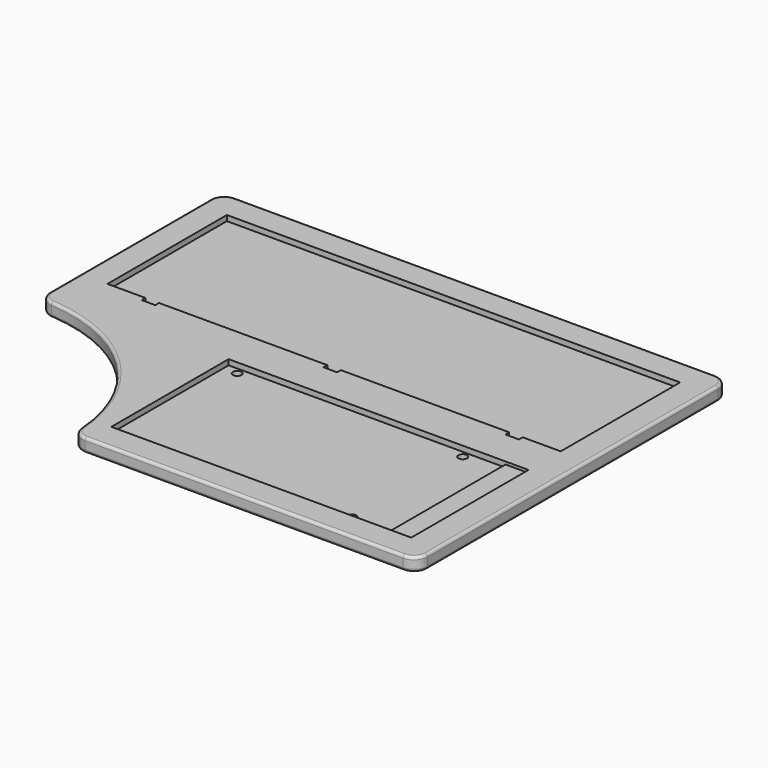
from build123d import *

# Parameters (mm, degrees)
F1_DEPTH = 5
F0_W     = 102
F0_H     = 54
F0_R     = 1.6
F2_DEPTH = 3
F0_W_2   = 8.5
F3_DEPTH = 4
F4_R     = 5
F5_R     = 1


with BuildPart() as f1:
    # F0 (on Top) → F1 (new body)
    with BuildSketch(Plane.XY):
        with BuildLine():
            Line((93.8627476096, 86.3866787127), (-93.1372523904, 86.3866787127))
            Line((-93.1372523904, 86.3866787127), (-93.1372523904, 2.5552856157))
            ThreePointArc((-93.1372523904, 2.5552856157), (-50.7122317842, -15.0177333034), (-33.1392128652, -57.4427539095))
            Line((-33.1392128652, -57.4427539095), (93.8627476096, -57.4427539095))
            Line((93.8627476096, -57.4427539095), (93.8627476096, 86.3866787127))
        make_face()
        Polygon((-26.6372523904, -47.4427539095), (-26.6372523904, 6.5572460905), (75.3627476096, 6.5572460905), (83.8627476096, 6.5572460905), (83.8627476096, -47.4427539095), (75.3627476096, -47.4427539095), align=None, mode=Mode.SUBTRACT)
        Polygon((-83.1372523904, 21.3866787127), (-83.1372523904, 76.3866787127), (83.8627476096, 76.3866787127), (83.8627476096, 21.3866787127), (69.8627476096, 21.3866787127), (69.8627476096, 19.6525212377), (64.8627476096, 19.6525212377), (64.8627476096, 21.3866787127), (2.8627476096, 21.3866787127), (2.8627476096, 19.6525212377), (-2.1372523904, 19.6525212377), (-2.1372523904, 21.3866787127), (-64.1372523904, 21.3866787127), (-64.1372523904, 19.6525212377), (-69.1372523904, 19.6525212377), (-69.1372523904, 21.3866787127), align=None, mode=Mode.SUBTRACT)
    extrude(amount=F1_DEPTH)

    # F0 (on Top) → F2 (join)
    with BuildSketch(Plane.XY):
        Polygon((83.8627476096, 76.3866787127), (-83.1372523904, 76.3866787127), (-83.1372523904, 21.3866787127), (-69.1372523904, 21.3866787127), (-69.1372523904, 19.6525212377), (-64.1372523904, 19.6525212377), (-64.1372523904, 21.3866787127), (-2.1372523904, 21.3866787127), (-2.1372523904, 19.6525212377), (2.8627476096, 19.6525212377), (2.8627476096, 21.3866787127), (64.8627476096, 21.3866787127), (64.8627476096, 19.6525212377), (69.8627476096, 19.6525212377), (69.8627476096, 21.3866787127), (83.8627476096, 21.3866787127), align=None)
        with Locations((24.3627476096, -20.4427539095)):
            Rectangle(F0_W, F0_H)
        with Locations((-21.5372523904, 4.1572460905)):
            Circle(F0_R, mode=Mode.SUBTRACT)
        with Locations((60.0627476096, -45.0427539095)):
            Circle(F0_R, mode=Mode.SUBTRACT)
        with Locations((61.5627476096, 4.1572460905)):
            Circle(F0_R, mode=Mode.SUBTRACT)
    extrude(amount=F2_DEPTH)

    # F0 (on Top) → F3 (join)
    with BuildSketch(Plane.XY):
        with Locations((79.6127476096, -20.4427539095)):
            Rectangle(F0_W_2, F0_H)
    extrude(amount=F3_DEPTH)

    # F4
    f4_edges = [f1.edges().sort_by_distance(p)[0] for p in [
        (93.862748, -57.442754, 2.5),
        (93.862748, 86.386679, 2.5),
        (-93.137252, 86.386679, 2.5),
        (-33.139213, -57.442754, 2.5),
        (-93.137252, 2.555286, 2.5),
    ]]
    fillet(f4_edges, radius=F4_R)

    # F5
    f5_edges = [f1.edges().sort_by_distance(p)[0] for p in [
        (93.862748, 14.471962, 5),
        (93.862748, 14.471962, 0),
        (92.398282, -55.978288, 0),
        (92.398282, 84.922213, 0),
        (30.265468, -57.442754, 0),
        (0.362748, 86.386679, 0),
        (-31.728639, -56.111755, 0),
        (-91.672786, 84.922213, 0),
        (-50.712232, -15.017733, 0),
        (-93.137252, 44.374683, 0),
        (-91.806253, 3.96586, 0),
        (59.962748, 4.157246, 0),
        (-23.137252, 4.157246, 0),
        (58.462748, -45.042754, 0),
        (92.398282, -55.978288, 5),
        (92.398282, 84.922213, 5),
        (30.265468, -57.442754, 5),
        (0.362748, 86.386679, 5),
        (-31.728639, -56.111755, 5),
        (-91.672786, 84.922213, 5),
        (-50.712232, -15.017733, 5),
        (-93.137252, 44.374683, 5),
        (-91.806253, 3.96586, 5),
    ]]
    fillet(f5_edges, radius=F5_R)


solid = f1.part
